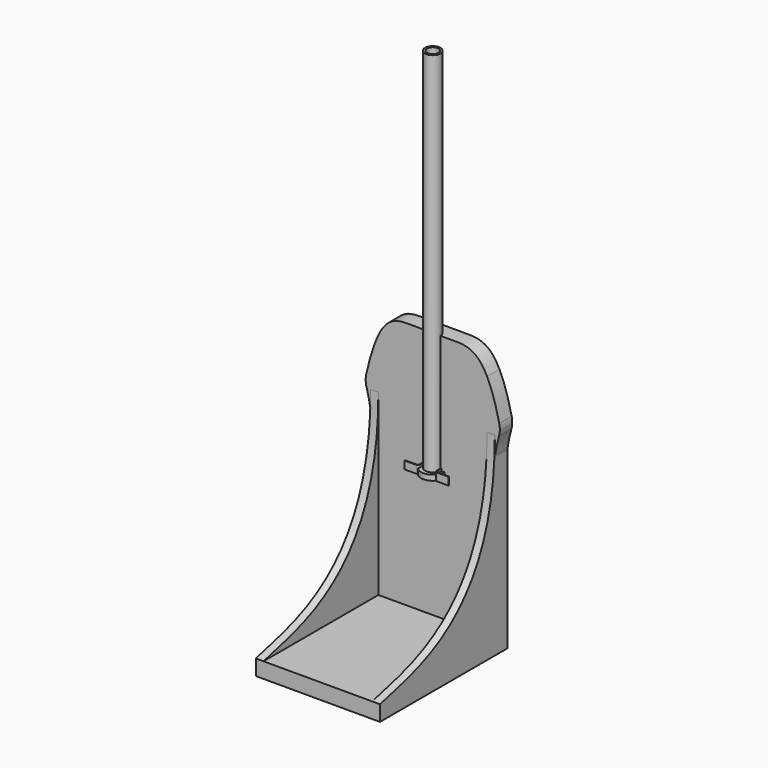
from build123d import *

# Parameters (mm, degrees)
F0_R      = 25.4
F0_R_2    = 19.05
F1_DEPTH  = 1219.2
F2_DEPTH  = 25.4
F4_DEPTH  = 17.4752
F6_D      = 7.62
F6_DEPTH  = 38.101
F7_D      = 7.62
F8_W      = 355.6
F8_H      = 50.8
F9_DEPTH  = 50.8
F11_DEPTH = 469.9
F12_DEPTH = 25.4
F14_DEPTH = 25.4
F15_DEPTH = 25.4


with BuildPart() as f1:
    # F0 (on Top) → F1 (new body)
    with BuildSketch(Plane.XY):
        Circle(F0_R)
        Circle(F0_R_2, mode=Mode.SUBTRACT)
    extrude(amount=F1_DEPTH)


with BuildPart() as f2:
    # F0 (on Top) → F2 (new body)
    with BuildSketch(Plane.XY):
        with BuildLine():
            Line((-26.9875, -19.05), (-26.9875, 0))
            ThreePointArc((-26.9875, 0), (0, 26.9875), (26.9875, 0))
            Line((26.9875, 0), (26.9875, -19.05))
            ThreePointArc((26.9875, -19.05), (28.8473719395, -23.5401280605), (33.3375, -25.4))
            Line((33.3375, -25.4), (71.4375, -25.4))
            Line((71.4375, -25.4), (71.4375, -23.1570992619))
            Line((71.4375, -23.1570992619), (33.3375, -23.1570992619))
            ThreePointArc((33.3375, -23.1570992619), (30.4333422609, -21.9541577391), (29.2304007381, -19.05))
            Line((29.2304007381, -19.05), (29.2304007381, 0))
            ThreePointArc((29.2304007381, 0), (0, 29.2304007381), (-29.2304007381, 0))
            Line((-29.2304007381, 0), (-29.2304007381, -19.05))
            ThreePointArc((-29.2304007381, -19.05), (-30.4333422609, -21.9541577391), (-33.3375, -23.1570992619))
            Line((-33.3375, -23.1570992619), (-71.4375, -23.1570992619))
            Line((-71.4375, -23.1570992619), (-71.4375, -25.4))
            Line((-71.4375, -25.4), (-33.3375, -25.4))
            ThreePointArc((-33.3375, -25.4), (-28.8473719395, -23.5401280605), (-26.9875, -19.05))
        make_face()
    extrude(amount=F2_DEPTH)


with BuildPart() as f4:
    # F3 (on Top) → F4 (new body)
    with BuildSketch(Plane.XY):
        with BuildLine():
            Line((-1.210663635, 25.3711311053), (-1.210663635, 38.0807601495))
            ThreePointArc((-1.210663635, 38.0807601495), (0, -38.1), (1.210663635, 38.0807601495))
            Line((1.210663635, 38.0807601495), (1.210663635, 25.3711311053))
            ThreePointArc((1.210663635, 25.3711311053), (0, -25.4), (-1.210663635, 25.3711311053))
        make_face()
    extrude(amount=F4_DEPTH)

    # F6 (through all, one way)
    with BuildSketch(Plane.YZ):
        with Locations((33.2899410278, 8.7780257373)):
            Circle(F6_D / 2)
    extrude(amount=-F6_DEPTH, mode=Mode.SUBTRACT)

    # F7 (through all)
    with Locations(Plane(origin=(0, 0, 0), x_dir=(0, 1, 0), z_dir=(-1, 0, 0))):
        with Locations((33.2899410278, -8.7780257373)):
            Hole(F7_D / 2)


with BuildPart() as f9:
    # F8 (on Front) → F9 (new body)
    with BuildSketch(Plane.XZ):
        with BuildLine():
            add(Edge.make_bspline(
                [(-10.5840112569, 406.4), (14.3579992132, 406.4), (84.774969433, 406.4), (143.8927068177, 406.4), (177.8, 338.6991968772)],
                knots=[0.4890074401, 0.4890074401, 0.4890074401, 0.4890074401, 0.6309879631, 0.8835658569, 0.8835658569, 0.8835658569, 0.8835658569], degree=3))
            add(Edge.make_bspline(
                [(-177.8, 342.347117997), (-146.667200487, 406.4), (-96.3951234553, 406.4), (-32.4144817487, 406.4), (-10.5840112569, 406.4)],
                knots=[0.1196529721, 0.1196529721, 0.1196529721, 0.1196529721, 0.364739125, 0.4890074401, 0.4890074401, 0.4890074401, 0.4890074401], degree=3))
            Line((-177.8, 342.347117997), (-177.8, 195.2799856663))
            Line((-177.8, 195.2799856663), (0, 195.2799856663))
            Line((0, 195.2799856663), (177.8, 195.2799856663))
            Line((177.8, 195.2799856663), (177.8, 338.6991968772))
        make_face()
        with BuildLine():
            add(Edge.make_bspline(
                [(177.8, 338.6991968772), (191.7201419538, 310.905625011), (204.9767238239, 271.7018098175), (217.617713139, 216.4034432339)],
                knots=[0.8835658569, 0.8835658569, 0.8835658569, 0.8835658569, 0.987258007, 0.987258007, 0.987258007, 0.987258007], degree=3))
            Line((177.8, 338.6991968772), (177.8, 195.2799856663))
            Line((177.8, 195.2799856663), (219.4212105721, 195.2799856663))
            ThreePointArc((219.4212105721, 195.2799856663), (219.2576697661, 205.9047418246), (217.617713139, 216.4034432339))
        make_face()
        with BuildLine():
            Line((-177.8, 195.2799856663), (-177.8, 342.347117997))
            add(Edge.make_bspline(
                [(-217.5700060395, 216.7215468508), (-204.5258308337, 274.3135632336), (-191.3744497579, 314.4189315762), (-177.8, 342.347117997)],
                knots=[0.0127910862, 0.0127910862, 0.0127910862, 0.0127910862, 0.1196529721, 0.1196529721, 0.1196529721, 0.1196529721], degree=3))
            ThreePointArc((-217.5700060395, 216.7215468508), (-219.2018900162, 206.0625792295), (-219.3128499865, 195.2799856663))
            Line((-219.3128499865, 195.2799856663), (-177.8, 195.2799856663))
        make_face()
        with BuildLine():
            Line((219.4212105721, 195.2799856663), (177.8, 195.2799856663))
            Line((177.8, 195.2799856663), (177.8, -406.4))
            add(Edge.make_bspline(
                [(216.4032871844, 177.8052482541), (179.1187861214, 51.7780463516), (191.9249839566, -215.2026964108), (177.8, -406.4)],
                knots=[28.1646192279, 28.1646192279, 28.1646192279, 28.1646192279, 603.319656278, 603.319656278, 603.319656278, 603.319656278], degree=3))
            ThreePointArc((216.4032871844, 177.8052482541), (218.4223260439, 186.454525576), (219.4212105721, 195.2799856663))
        make_face()
        Polygon((177.8, -406.4), (177.8, 195.2799856663), (0, 195.2799856663), (-177.8, 195.2799856663), (-177.8, -406.4), align=None)
        with BuildLine():
            Line((-177.8, -406.4), (-177.8, 195.2799856663))
            Line((-177.8, 195.2799856663), (-219.3128499865, 195.2799856663))
            ThreePointArc((-219.3128499865, 195.2799856663), (-218.2545301806, 186.4311737852), (-216.1703176559, 177.76644236))
            add(Edge.make_bspline(
                [(-216.1703176559, 177.76644236), (-179.1721643238, 55.8179762585), (-191.8954816103, -215.602043346), (-177.8, -406.4)],
                knots=[29.3659248791, 29.3659248791, 29.3659248791, 29.3659248791, 603.319656278, 603.319656278, 603.319656278, 603.319656278], degree=3))
        make_face()
        with Locations((0, -431.8)):
            Rectangle(F8_W, F8_H)
    extrude(amount=-F9_DEPTH)

    # F8 (on Front) → F11 (join)
    with BuildSketch(Plane.XZ):
        with Locations((0, -431.8)):
            Rectangle(F8_W, F8_H)
    extrude(amount=F11_DEPTH)

    # F12 (add, symmetric): faces of the model
    f12_faces = [f9.faces().sort_by_distance(p)[0] for p in [
        (177.8, -209.55, -431.8),
        (-177.8, -209.55, -431.8),
    ]]
    extrude(f12_faces, amount=F12_DEPTH, both=True, dir=(1, 0, 0))

    # F10 (on face) → F14 (join)
    with BuildSketch(Plane.YZ.offset(177.8)):
        with BuildLine():
            Line((50.8, 177.7829378843), (0, 177.7829378843))
            add(Edge.make_bspline(
                [(0, 177.7829378843), (0, -337.2519960899), (-327.5773703098, -367.0474041939), (-469.9, -406.4)],
                knots=[0, 0, 0, 0, 749.717089918, 749.717089918, 749.717089918, 749.717089918], degree=3))
            Line((-469.9, -406.4), (50.8, -406.4))
            Line((50.8, -406.4), (50.8, 177.7829378843))
        make_face()
    extrude(amount=F14_DEPTH)

    # F13 (on face) → F15 (join)
    with BuildSketch(Plane(origin=(-203.2, 0, 0), x_dir=(0, -1, 0), z_dir=(-1, 0, 0))):
        with BuildLine():
            Line((0, 177.2581189871), (-50.8, 177.2581189871))
            Line((-50.8, 177.2581189871), (-50.8, -406.4))
            Line((-50.8, -406.4), (469.9, -406.4))
            add(Edge.make_bspline(
                [(0, 177.2581189871), (0, -337.4345749617), (327.5773703098, -367.0474041939), (469.9, -406.4)],
                knots=[0, 0, 0, 0, 749.3082208674, 749.3082208674, 749.3082208674, 749.3082208674], degree=3))
        make_face()
    extrude(amount=-F15_DEPTH)


solid = Compound([f1.part, f2.part, f4.part, f9.part])
